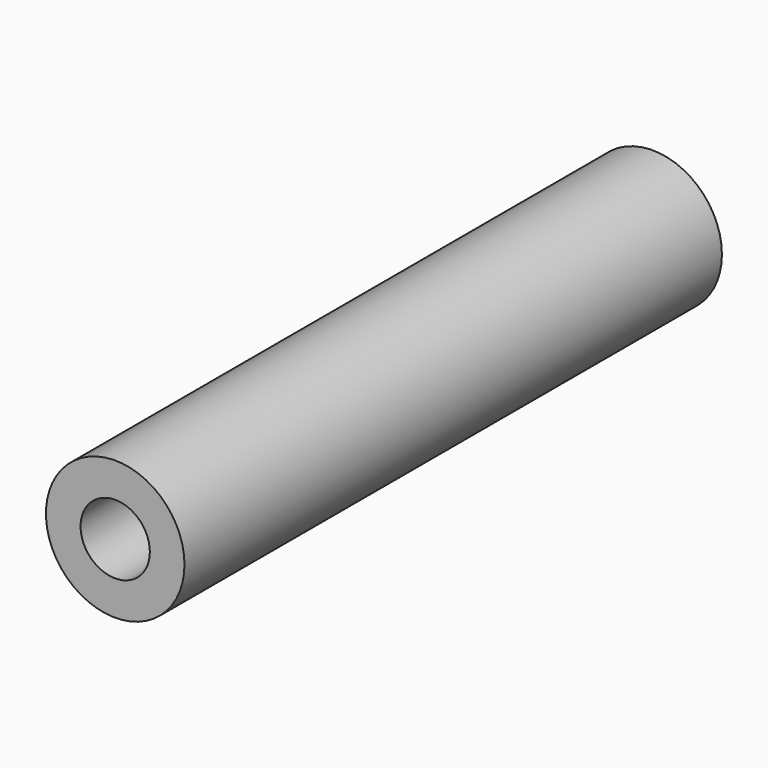
from build123d import *

# Parameters (mm, degrees)
F0_R     = 20
F0_R_2   = 10
F1_DEPTH = 194


# Not quite as in the source:
# - a feature names something its author has since deleted; it is built from what else it names


with BuildPart() as f1:
    # F0 (on Front) → F1 (new body)
    with BuildSketch(Plane.XZ):
        Circle(F0_R)
        Circle(F0_R_2, mode=Mode.SUBTRACT)
    extrude(amount=F1_DEPTH)


solid = f1.part
